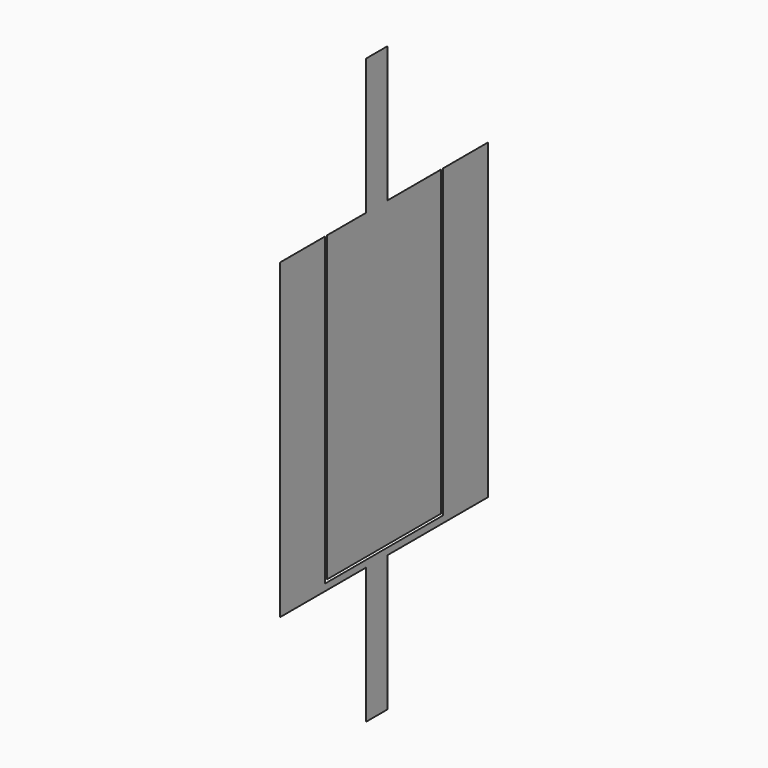
from build123d import *

# Parameters (mm, degrees)
F1_DEPTH = 0.0012


# Not quite as in the source:
# - a feature names something its author has since deleted; it is built from what else it names


with BuildPart() as f1:
    # F0 (on Right) → F1 (new body)
    with BuildSketch(Plane.YZ):
        Polygon((6.5217, 0), (0, 0), (0, -60), (12, -60), (12.4011761725, -60), (20.65, -60), (20.65, -86.0869), (25.87, -86.0869), (25.87, -81.0653850647), (25.87, -60), (50, -60), (50, 0), (39.131, 0), (39.131, -27.64149), (39.131, -58.696), (10.8695, -58.696), (10.8695, -27.64149), (10.8695, 0), (9, 0), align=None)
    extrude(amount=F1_DEPTH)


with BuildPart() as f1b:
    # F0 (on Right) → F1, piece 2 (new body)
    with BuildSketch(Plane.YZ):
        Polygon((16.08474, 0), (11.4456, 0), (11.36984, 0), (11.36984, -26.73915), (11.36984, -27.14115), (11.36984, -58.196), (38.63066, -58.196), (38.63066, -27.14115), (38.63066, -26.73915), (38.63066, 0), (25.87, 0), (25.87, 26.0869), (20.65, 26.0869), (20.65, 0), align=None)
    extrude(amount=F1_DEPTH)


solid = Compound([f1.part, f1b.part])
